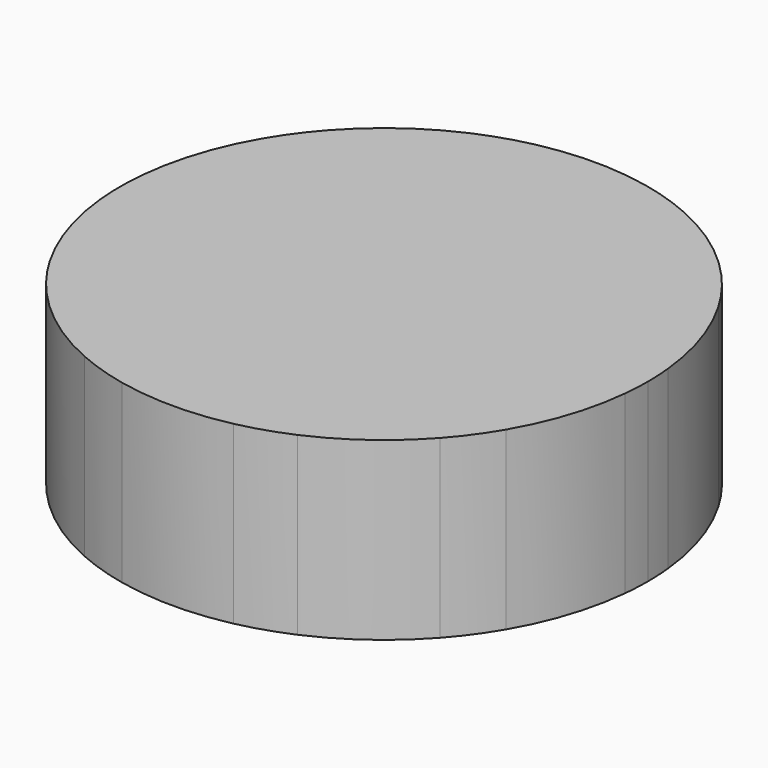
from build123d import *

# Parameters (mm, degrees)
F1_DEPTH = 25.4


# Not quite as in the source:
# - a feature names something its author has since deleted; it is built from what else it names


with BuildPart() as f1:
    # F0 (on Top) → F1 (new body)
    with BuildSketch(Plane.XY):
        with BuildLine():
            ThreePointArc((-13.8407698917, 49.932215552), (-13.693941355, 51.8586333583), (-13.6449565232, 53.7900174916))
            ThreePointArc((-13.6449565232, 53.7900174916), (-13.693941355, 55.7214016248), (-13.8407698917, 57.6478194312))
            ThreePointArc((-13.8407698917, 57.6478194312), (-15.5097032523, 65.5635649773), (-18.812266294, 72.9485120636))
            ThreePointArc((-18.812266294, 72.9485120636), (-20.9214090375, 76.1846356039), (-23.3473844667, 79.1905667238))
            ThreePointArc((-23.3473844667, 79.1905667238), (-29.3503384108, 84.6135649773), (-36.3629310228, 88.6469148221))
            ThreePointArc((-36.3629310228, 88.6469148221), (-39.9714090375, 90.0252707624), (-43.7009063693, 91.0311675426))
            ThreePointArc((-43.7009063693, 91.0311675426), (-51.7449565232, 91.8900174916), (-59.789006677, 91.0311675426))
            ThreePointArc((-59.789006677, 91.0311675426), (-63.5185040089, 90.0252707624), (-67.1269820235, 88.6469148221))
            ThreePointArc((-67.1269820235, 88.6469148221), (-74.1395746355, 84.6135649773), (-80.1425285796, 79.1905667238))
            ThreePointArc((-80.1425285796, 79.1905667238), (-82.5685040089, 76.1846356039), (-84.6776467524, 72.9485120636))
            ThreePointArc((-84.6776467524, 72.9485120636), (-87.980209794, 65.5635649773), (-89.6491431547, 57.6478194312))
            ThreePointArc((-89.6491431547, 57.6478194312), (-89.8449565232, 53.7900174916), (-89.6491431547, 49.932215552))
            ThreePointArc((-89.6491431547, 49.932215552), (-87.980209794, 42.0164700059), (-84.6776467524, 34.6315229195))
            ThreePointArc((-84.6776467524, 34.6315229195), (-82.5685040089, 31.3953993792), (-80.1425285796, 28.3894682594))
            ThreePointArc((-80.1425285796, 28.3894682594), (-74.1395746355, 22.9664700059), (-67.1269820235, 18.9331201611))
            ThreePointArc((-67.1269820235, 18.9331201611), (-63.5185040089, 17.5547642207), (-59.789006677, 16.5488674406))
            ThreePointArc((-59.789006677, 16.5488674406), (-51.7449565232, 15.6900174916), (-43.7009063693, 16.5488674406))
            ThreePointArc((-43.7009063693, 16.5488674406), (-39.9714090375, 17.5547642207), (-36.3629310228, 18.9331201611))
            ThreePointArc((-36.3629310228, 18.9331201611), (-29.3503384108, 22.9664700059), (-23.3473844667, 28.3894682594))
            ThreePointArc((-23.3473844667, 28.3894682594), (-20.9214090375, 31.3953993792), (-18.812266294, 34.6315229195))
            ThreePointArc((-18.812266294, 34.6315229195), (-15.5097032523, 42.0164700059), (-13.8407698917, 49.932215552))
        make_face()
    extrude(amount=F1_DEPTH)


solid = f1.part
